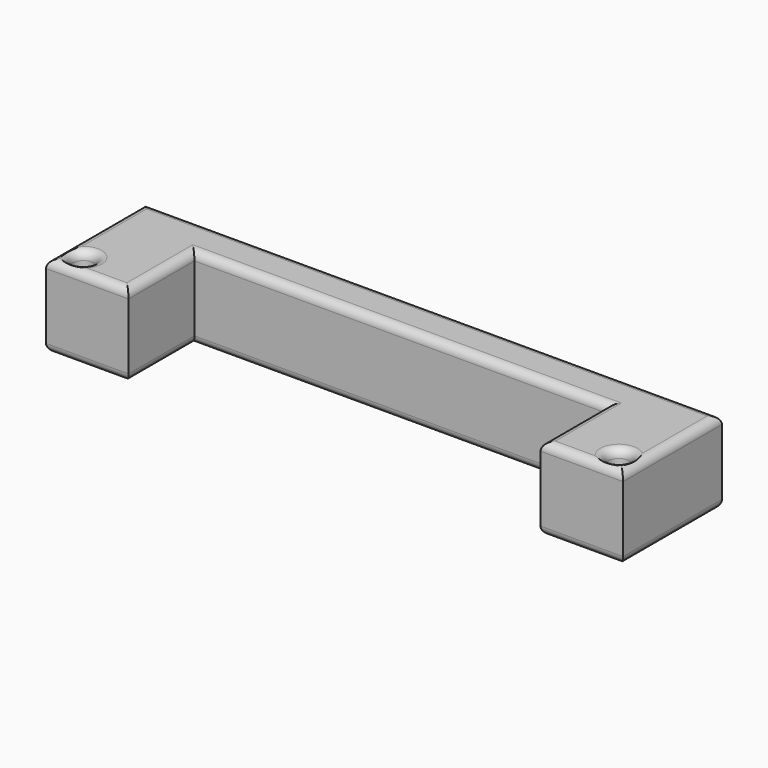
from build123d import *

# Parameters (mm, degrees)
F1_DEPTH     = 20
F3_D         = 5
F5_T3_DEPTH  = 150
F5_T6_DEPTH  = 40
F5_T9_DEPTH  = 30
F5_T12_DEPTH = 25
F5_T15_DEPTH = 100
F5_T18_DEPTH = 25
F5_T21_DEPTH = 30
F5_T24_DEPTH = 40
F5_T33_DEPTH = 150
F5_T36_DEPTH = 40
F5_T39_DEPTH = 30
F5_T42_DEPTH = 25
F5_T45_DEPTH = 100
F5_T48_DEPTH = 25
F5_T51_DEPTH = 30
F5_T54_DEPTH = 40
F5_T64_DEPTH = 105
F5_T68_DEPTH = 30
F5_T74_DEPTH = 30
F5_T78_DEPTH = 105
F5_T84_DEPTH = 30
F5_T88_DEPTH = 105
F5_T94_DEPTH = 105
F5_T98_DEPTH = 30


# Not quite as in the source:
# - a fillet or chamfer that OpenCascade refuses, or shapes differently, is made with other operations: its cross-section is extruded or revolved along the edge and cut away or added


with BuildPart() as f1:
    # F0 (on Top) → F1 (new body)
    with BuildSketch(Plane.XY):
        Polygon((45.4953936456, 30), (-24.5046063544, 30), (-24.5046063544, 20), (25.4953936456, 20), (25.4953936456, 0), (45.4953936456, 0), align=None)
    extrude(amount=F1_DEPTH)

    # F3 (through all)
    with Locations(Plane.XY.offset(20)):
        with Locations((40.4953936456, 5)):
            Hole(F3_D / 2)

    # F4: F1 across face


with BuildPart() as f1_1:
    add(f1.part)
    add(f1.part.mirror(Plane(origin=(-24.5046063544, 25, 10), x_dir=(0, -1, 0), z_dir=(-1, 0, 0))))

    # F5: fillet of radius 2 on 20 edges, made by hand


with BuildPart() as f5_tool1:
    # F5_s2 → F5_t3 (new body)
    with BuildSketch(Plane.YZ.offset(-99.5046063544)):
        with BuildLine():
            ThreePointArc((30, 18), (29.4142135624, 19.4142135624), (28, 20))
            Line((28, 20), (30, 20))
            Line((30, 20), (30, 18))
        make_face()
    extrude(amount=F5_T3_DEPTH)


with BuildPart() as f5_tool4:
    # F5_s5 → F5_t6 (new body)
    with BuildSketch(Plane.XZ.offset(5)):
        with BuildLine():
            ThreePointArc((-94.5046063544, 18), (-93.9188199167, 19.4142135624), (-92.5046063544, 20))
            Line((-92.5046063544, 20), (-94.5046063544, 20))
            Line((-94.5046063544, 20), (-94.5046063544, 18))
        make_face()
    extrude(amount=-F5_T6_DEPTH)


with BuildPart() as f5_tool7:
    # F5_s8 → F5_t9 (new body)
    with BuildSketch(Plane.YZ.offset(-69.5046063544)):
        with BuildLine():
            ThreePointArc((0, 18), (0.5857864376, 19.4142135624), (2, 20))
            Line((2, 20), (0, 20))
            Line((0, 20), (0, 18))
        make_face()
    extrude(amount=-F5_T9_DEPTH)


with BuildPart() as f5_tool10:
    # F5_s11 → F5_t12 (new body)
    with BuildSketch(Plane.XZ.offset(-20)):
        with BuildLine():
            ThreePointArc((-74.5046063544, 18), (-75.090392792, 19.4142135624), (-76.5046063544, 20))
            Line((-76.5046063544, 20), (-74.5046063544, 20))
            Line((-74.5046063544, 20), (-74.5046063544, 18))
        make_face()
    extrude(amount=F5_T12_DEPTH)


with BuildPart() as f5_tool13:
    # F5_s14 → F5_t15 (new body)
    with BuildSketch(Plane.YZ.offset(-74.5046063544)):
        with BuildLine():
            ThreePointArc((20, 18), (20.5857864376, 19.4142135624), (22, 20))
            Line((22, 20), (20, 20))
            Line((20, 20), (20, 18))
        make_face()
    extrude(amount=F5_T15_DEPTH)


with BuildPart() as f5_tool16:
    # F5_s17 → F5_t18 (new body)
    with BuildSketch(Plane.XZ.offset(-20)):
        with BuildLine():
            ThreePointArc((25.4953936456, 18), (26.0811800833, 19.4142135624), (27.4953936456, 20))
            Line((27.4953936456, 20), (25.4953936456, 20))
            Line((25.4953936456, 20), (25.4953936456, 18))
        make_face()
    extrude(amount=F5_T18_DEPTH)


with BuildPart() as f5_tool19:
    # F5_s20 → F5_t21 (new body)
    with BuildSketch(Plane.YZ.offset(20.4953936456)):
        with BuildLine():
            ThreePointArc((0, 18), (0.5857864376, 19.4142135624), (2, 20))
            Line((2, 20), (0, 20))
            Line((0, 20), (0, 18))
        make_face()
    extrude(amount=F5_T21_DEPTH)


with BuildPart() as f5_tool22:
    # F5_s23 → F5_t24 (new body)
    with BuildSketch(Plane.XZ.offset(5)):
        with BuildLine():
            ThreePointArc((43.4953936456, 20), (44.909607208, 19.4142135624), (45.4953936456, 18))
            Line((45.4953936456, 18), (45.4953936456, 20))
            Line((45.4953936456, 20), (43.4953936456, 20))
        make_face()
    extrude(amount=-F5_T24_DEPTH)


with BuildPart() as f5_tool25:
    # F5_s26 → F5_t27 (revolve)
    with BuildSketch(Plane.XZ.offset(-5)):
        with BuildLine():
            ThreePointArc((42.9953936456, 18), (43.5811800833, 19.4142135624), (44.9953936456, 20))
            Line((44.9953936456, 20), (42.9953936456, 20))
            Line((42.9953936456, 20), (42.9953936456, 18))
        make_face()
    revolve(axis=Axis((40.4953936456, 5, 20), (0, 0, 1)))


with BuildPart() as f5_tool28:
    # F5_s29 → F5_t30 (revolve)
    with BuildSketch(Plane.XZ.offset(-5)):
        with BuildLine():
            ThreePointArc((-92.0046063544, 18), (-92.590392792, 19.4142135624), (-94.0046063544, 20))
            Line((-94.0046063544, 20), (-92.0046063544, 20))
            Line((-92.0046063544, 20), (-92.0046063544, 18))
        make_face()
    revolve(axis=Axis((-89.5046063544, 5, 20), (0, 0, -1)))


with BuildPart() as f5_tool31:
    # F5_s32 → F5_t33 (new body)
    with BuildSketch(Plane.YZ.offset(50.4953936456)):
        with BuildLine():
            ThreePointArc((30, 2), (29.4142135624, 0.5857864376), (28, 0))
            Line((28, 0), (30, 0))
            Line((30, 0), (30, 2))
        make_face()
    extrude(amount=-F5_T33_DEPTH)


with BuildPart() as f5_tool34:
    # F5_s35 → F5_t36 (new body)
    with BuildSketch(Plane.XZ.offset(5)):
        with BuildLine():
            ThreePointArc((-92.5046063544, 0), (-93.9188199167, 0.5857864376), (-94.5046063544, 2))
            Line((-94.5046063544, 2), (-94.5046063544, 0))
            Line((-94.5046063544, 0), (-92.5046063544, 0))
        make_face()
    extrude(amount=-F5_T36_DEPTH)


with BuildPart() as f5_tool37:
    # F5_s38 → F5_t39 (new body)
    with BuildSketch(Plane.YZ.offset(-69.5046063544)):
        with BuildLine():
            ThreePointArc((2, 0), (0.5857864376, 0.5857864376), (0, 2))
            Line((0, 2), (0, 0))
            Line((0, 0), (2, 0))
        make_face()
    extrude(amount=-F5_T39_DEPTH)


with BuildPart() as f5_tool40:
    # F5_s41 → F5_t42 (new body)
    with BuildSketch(Plane.XZ.offset(-20)):
        with BuildLine():
            ThreePointArc((-76.5046063544, 0), (-75.090392792, 0.5857864376), (-74.5046063544, 2))
            Line((-74.5046063544, 2), (-74.5046063544, 0))
            Line((-74.5046063544, 0), (-76.5046063544, 0))
        make_face()
    extrude(amount=F5_T42_DEPTH)


with BuildPart() as f5_tool43:
    # F5_s44 → F5_t45 (new body)
    with BuildSketch(Plane.YZ.offset(25.4953936456)):
        with BuildLine():
            ThreePointArc((22, 0), (20.5857864376, 0.5857864376), (20, 2))
            Line((20, 2), (20, 0))
            Line((20, 0), (22, 0))
        make_face()
    extrude(amount=-F5_T45_DEPTH)


with BuildPart() as f5_tool46:
    # F5_s47 → F5_t48 (new body)
    with BuildSketch(Plane.XZ.offset(-20)):
        with BuildLine():
            ThreePointArc((27.4953936456, 0), (26.0811800833, 0.5857864376), (25.4953936456, 2))
            Line((25.4953936456, 2), (25.4953936456, 0))
            Line((25.4953936456, 0), (27.4953936456, 0))
        make_face()
    extrude(amount=F5_T48_DEPTH)


with BuildPart() as f5_tool49:
    # F5_s50 → F5_t51 (new body)
    with BuildSketch(Plane.YZ.offset(20.4953936456)):
        with BuildLine():
            ThreePointArc((2, 0), (0.5857864376, 0.5857864376), (0, 2))
            Line((0, 2), (0, 0))
            Line((0, 0), (2, 0))
        make_face()
    extrude(amount=F5_T51_DEPTH)


with BuildPart() as f5_tool52:
    # F5_s53 → F5_t54 (new body)
    with BuildSketch(Plane.XZ.offset(5)):
        with BuildLine():
            ThreePointArc((43.4953936456, 0), (44.909607208, 0.5857864376), (45.4953936456, 2))
            Line((45.4953936456, 2), (45.4953936456, 0))
            Line((45.4953936456, 0), (43.4953936456, 0))
        make_face()
    extrude(amount=-F5_T54_DEPTH)


with BuildPart() as f5_tool55:
    # F5_s56 → F5_t57 (revolve)
    with BuildSketch(Plane.XZ.offset(-5)):
        with BuildLine():
            ThreePointArc((44.9953936456, 0), (43.5811800833, 0.5857864376), (42.9953936456, 2))
            Line((42.9953936456, 2), (42.9953936456, 0))
            Line((42.9953936456, 0), (44.9953936456, 0))
        make_face()
    revolve(axis=Axis((40.4953936456, 5, 0), (0, 0, 1)))


with BuildPart() as f5_tool58:
    # F5_s59 → F5_t60 (revolve)
    with BuildSketch(Plane.XZ.offset(-5)):
        with BuildLine():
            ThreePointArc((-94.0046063544, 0), (-92.590392792, 0.5857864376), (-92.0046063544, 2))
            Line((-92.0046063544, 2), (-92.0046063544, 0))
            Line((-92.0046063544, 0), (-94.0046063544, 0))
        make_face()
    revolve(axis=Axis((-89.5046063544, 5, 0), (0, 0, -1)))


with BuildPart() as f5_tool62:
    # F5_s63 → F5_t64 (new body)
    with BuildSketch(Plane.YZ.offset(-79.5046063544)):
        with BuildLine():
            ThreePointArc((20, 18), (20.5857864376, 19.4142135624), (22, 20))
            Line((22, 20), (20, 20))
            Line((20, 20), (20, 18))
        make_face()
    extrude(amount=F5_T64_DEPTH)

    split(bisect_by=Plane.YZ.offset(-74.5046063544), keep=Keep.BOTTOM)


with BuildPart() as f5_tool66:
    # F5_s67 → F5_t68 (new body)
    with BuildSketch(Plane.XZ.offset(-25)):
        with BuildLine():
            ThreePointArc((-74.5046063544, 18), (-75.090392792, 19.4142135624), (-76.5046063544, 20))
            Line((-76.5046063544, 20), (-74.5046063544, 20))
            Line((-74.5046063544, 20), (-74.5046063544, 18))
        make_face()
    extrude(amount=F5_T68_DEPTH)

    split(bisect_by=Plane.XZ.offset(-20), keep=Keep.BOTTOM)


with BuildPart() as f5_tool62_1:
    add(f5_tool62.part)

    # F5_t70: intersect F5_tool66
    add(f5_tool66.part, mode=Mode.INTERSECT)


with BuildPart() as f5_tool72:
    # F5_s73 → F5_t74 (new body)
    with BuildSketch(Plane.XZ.offset(-25)):
        with BuildLine():
            ThreePointArc((25.4953936456, 18), (26.0811800833, 19.4142135624), (27.4953936456, 20))
            Line((27.4953936456, 20), (25.4953936456, 20))
            Line((25.4953936456, 20), (25.4953936456, 18))
        make_face()
    extrude(amount=F5_T74_DEPTH)

    split(bisect_by=Plane.XZ.offset(-20), keep=Keep.BOTTOM)


with BuildPart() as f5_tool76:
    # F5_s77 → F5_t78 (new body)
    with BuildSketch(Plane.YZ.offset(-74.5046063544)):
        with BuildLine():
            ThreePointArc((20, 18), (20.5857864376, 19.4142135624), (22, 20))
            Line((22, 20), (20, 20))
            Line((20, 20), (20, 18))
        make_face()
    extrude(amount=F5_T78_DEPTH)

    split(bisect_by=Plane.YZ.offset(25.4953936456), keep=Keep.TOP)


with BuildPart() as f5_tool72_1:
    add(f5_tool72.part)

    # F5_t80: intersect F5_tool76
    add(f5_tool76.part, mode=Mode.INTERSECT)


with BuildPart() as f5_tool82:
    # F5_s83 → F5_t84 (new body)
    with BuildSketch(Plane.XZ.offset(-25)):
        with BuildLine():
            ThreePointArc((-76.5046063544, 0), (-75.090392792, 0.5857864376), (-74.5046063544, 2))
            Line((-74.5046063544, 2), (-74.5046063544, 0))
            Line((-74.5046063544, 0), (-76.5046063544, 0))
        make_face()
    extrude(amount=F5_T84_DEPTH)

    split(bisect_by=Plane.XZ.offset(-20), keep=Keep.BOTTOM)


with BuildPart() as f5_tool86:
    # F5_s87 → F5_t88 (new body)
    with BuildSketch(Plane.YZ.offset(25.4953936456)):
        with BuildLine():
            ThreePointArc((22, 0), (20.5857864376, 0.5857864376), (20, 2))
            Line((20, 2), (20, 0))
            Line((20, 0), (22, 0))
        make_face()
    extrude(amount=-F5_T88_DEPTH)

    split(bisect_by=Plane.YZ.offset(-74.5046063544), keep=Keep.BOTTOM)


with BuildPart() as f5_tool82_1:
    add(f5_tool82.part)

    # F5_t90: intersect F5_tool86
    add(f5_tool86.part, mode=Mode.INTERSECT)


with BuildPart() as f5_tool92:
    # F5_s93 → F5_t94 (new body)
    with BuildSketch(Plane.YZ.offset(30.4953936456)):
        with BuildLine():
            ThreePointArc((22, 0), (20.5857864376, 0.5857864376), (20, 2))
            Line((20, 2), (20, 0))
            Line((20, 0), (22, 0))
        make_face()
    extrude(amount=-F5_T94_DEPTH)

    split(bisect_by=Plane.YZ.offset(25.4953936456), keep=Keep.TOP)


with BuildPart() as f5_tool96:
    # F5_s97 → F5_t98 (new body)
    with BuildSketch(Plane.XZ.offset(-25)):
        with BuildLine():
            ThreePointArc((27.4953936456, 0), (26.0811800833, 0.5857864376), (25.4953936456, 2))
            Line((25.4953936456, 2), (25.4953936456, 0))
            Line((25.4953936456, 0), (27.4953936456, 0))
        make_face()
    extrude(amount=F5_T98_DEPTH)

    split(bisect_by=Plane.XZ.offset(-20), keep=Keep.BOTTOM)


with BuildPart() as f5_tool92_1:
    add(f5_tool92.part)

    # F5_t100: intersect F5_tool96
    add(f5_tool96.part, mode=Mode.INTERSECT)


with BuildPart() as f1_2:
    add(f1_1.part)

    # F5_t101: cut F5_tool1, F5_tool4, F5_tool7, F5_tool10, F5_tool13, F5_tool16, F5_tool19, F5_tool22, F5_tool25, F5_tool28, F5_tool31, F5_tool34, F5_tool37, F5_tool40, F5_tool43, F5_tool46, F5_tool49, F5_tool52, F5_tool55, F5_tool58, F5_tool62, F5_tool72, F5_tool82, F5_tool92
    add([f5_tool1.part, f5_tool4.part, f5_tool7.part, f5_tool10.part, f5_tool13.part, f5_tool16.part, f5_tool19.part, f5_tool22.part, f5_tool25.part, f5_tool28.part, f5_tool31.part, f5_tool34.part, f5_tool37.part, f5_tool40.part, f5_tool43.part, f5_tool46.part, f5_tool49.part, f5_tool52.part, f5_tool55.part, f5_tool58.part, f5_tool62_1.part, f5_tool72_1.part, f5_tool82_1.part, f5_tool92_1.part], mode=Mode.SUBTRACT)


solid = f1_2.part
